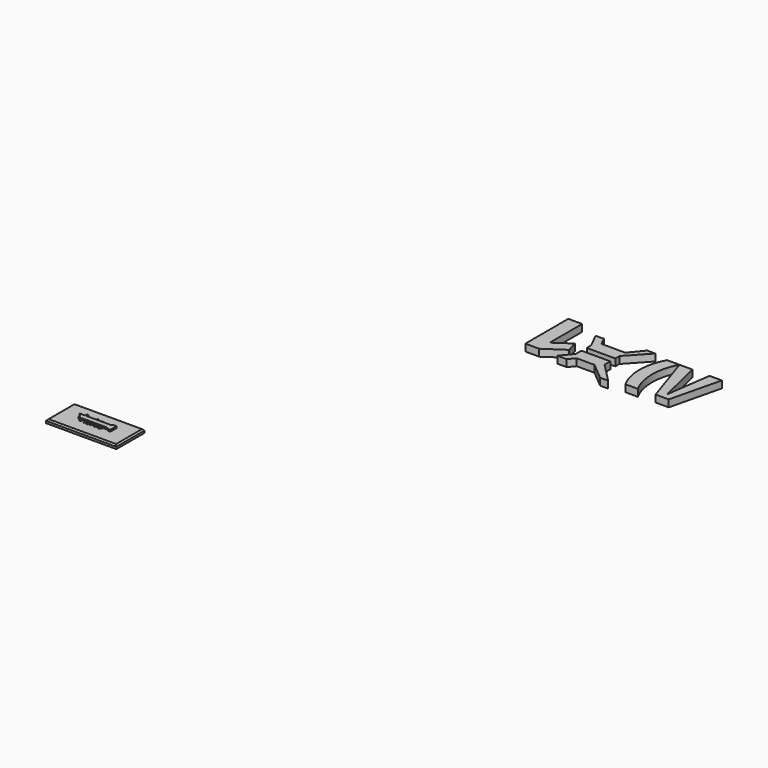
from build123d import *

# Parameters (mm, degrees)
F2_DEPTH      = 50.8
F0_W          = 208.8167369366
F0_H          = 51.5262037516
F0_W_2        = 205.8834665987
F0_H_2        = 38.4079218469
F4_DEPTH      = 50.8
F6_DEPTH      = 38.1
F7_W          = 508
F7_H          = 254
F8_DEPTH      = 25.4
F10_TEXT_SIZE = 24.7326162126
F9_TEXT_SIZE  = 38.4211540222
F11_DEPTH     = 25.4
F12_SIZE      = 10.16


# Not quite as in the source:
# - a feature names something its author has since deleted; it is built from what else it names
# - Text() gives the source's letters only with a copy of the font that has no kerning and outlines rounded to 1/6400 em; it was checked with that copy


with BuildPart() as f2:
    # F1 (on Top) → F2 (new body)
    with BuildSketch(Plane.XY):
        Polygon((1089.858174324, 166.3102060556), (997.6534247398, 166.3102060556), (1119.6892261505, -202.5089114904), (1214.6058082581, -202.5089114904), (1304.0987253189, 166.3102060556), (1214.6058082581, 166.3102060556), (1168.5034036636, -159.1184288263), align=None)
    extrude(amount=F2_DEPTH)


with BuildPart() as f2b:
    # F1 (on Top) → F2, piece 2 (new body)
    with BuildSketch(Plane.XY):
        with BuildLine():
            ThreePointArc((908.1605672836, 166.3102060556), (859.1155412482, -22.1672132611), (908.1605672836, -210.6446325779))
            Line((908.1605672836, -210.6446325779), (997.6534247398, -210.6446325779))
            ThreePointArc((997.6534247398, -210.6446325779), (949.8001223962, -22.1672132611), (997.6534247398, 166.3102060556))
            Line((997.6534247398, 166.3102060556), (908.1605672836, 166.3102060556))
        make_face()
    extrude(amount=F2_DEPTH)


with BuildPart() as f2c:
    # F0 (on Top) → F2, piece 3 (new body)
    with BuildSketch(Plane.XY):
        with Locations((562.3926073313, -70.981502533)):
            Rectangle(F0_W, F0_H)
        Polygon((666.8009757996, -96.7446044087), (457.984238863, -96.7446044087), (390.1866078377, -178.1017631292), (457.984238863, -178.1017631292), (494.6616488046, -134.0888703932), (623.4104633331, -134.0888703932), (747.2194167122, -237.2629963194), (805.1081299782, -237.2629963194), align=None)
    extrude(amount=F2_DEPTH)


with BuildPart() as f2d:
    # F0 (on Top) → F2, piece 4 (new body)
    with BuildSketch(Plane.XY):
        Polygon((406.4580502787, 147.3268717527), (460.9175092009, 38.4079218469), (666.8009757996, 38.4079218469), (805.1081299782, 188.0054622889), (747.2194167122, 188.0054622889), (666.8009757996, 90.376868844), (494.6616488046, 90.376868844), (466.1199748516, 147.3268717527), align=None)
        with Locations((563.8592425002, 19.2039609235)):
            Rectangle(F0_W_2, F0_H_2)
    extrude(amount=F2_DEPTH)


with BuildPart() as f4:
    # F3 (on Top) → F4 (new body)
    with BuildSketch(Plane.XY):
        Polygon((156.9627672434, 212.4126106501), (156.9627672434, -175.3898561001), (257.3032677174, -175.3898561001), (257.3032677174, -80.473177135), (257.3032677174, 212.4126106501), align=None)
        Polygon((257.3032677174, -80.473177135), (257.3032677174, -175.3898561001), (398.322314024, -80.473177135), (373.9151656628, 0), align=None)
    extrude(amount=F4_DEPTH)


with BuildPart() as f6:
    # F5 (on Top) → F6 (new body)
    with BuildSketch(Plane.XY):
        with BuildLine():
            Line((-1066.0594806806, -2393.8014631634), (-1240.2185239818, -2393.8014631634))
            Line((-1240.2185239818, -2393.8014631634), (-1240.2185239818, -2431.1765145333))
            Line((-1240.2185239818, -2431.1765145333), (-1066.0594806806, -2431.1765145333))
            Line((-1066.0594806806, -2431.1765145333), (-1061.7204306761, -2431.1765145333))
            ThreePointArc((-1061.7204306761, -2431.1765145333), (-1046.5276988746, -2440.3088155686), (-1028.8736676509, -2438.7109409353))
            Line((-1028.8736676509, -2438.7109409353), (-1028.8736676509, -2414.7824282699))
            Line((-1028.8736676509, -2414.7824282699), (-1028.8736676509, -2412.4889888483))
            Line((-1028.8736676509, -2412.4889888483), (-1028.8736676509, -2406.4367107859))
            Line((-1028.8736676509, -2406.4367107859), (-1028.8736676509, -2403.9940772423))
            Line((-1028.8736676509, -2403.9940772423), (-1028.8736676509, -2396.0567906488))
            Line((-1028.8736676509, -2396.0567906488), (-1028.8736676509, -2393.8014631634))
            Line((-1028.8736676509, -2393.8014631634), (-1028.8736676509, -2386.2670367614))
            ThreePointArc((-1028.8736676509, -2386.2670367614), (-1046.5276988746, -2384.6691621281), (-1061.7204306761, -2393.8014631634))
            Line((-1061.7204306761, -2393.8014631634), (-1066.0594806806, -2393.8014631634))
        make_face()
        Polygon((-1248.5956841506, -2430.5321082507), (-1248.5956841506, -2406.7832553444), (-1269.2164084326, -2406.7832553444), (-1269.2164084326, -2411.8445825658), align=None)
        Polygon((-1248.5956841506, -2406.7832553444), (-1248.5956841506, -2393.6926673954), (-1289.8371327145, -2393.1570568808), (-1269.2164084326, -2411.8445825658), (-1269.2164084326, -2406.7832553444), align=None)
        Polygon((-1240.2185239818, -2431.1765145333), (-1240.2185239818, -2393.8014631634), (-1248.5956841506, -2393.6926673954), (-1248.5956841506, -2406.7832553444), (-1248.5956841506, -2430.5321082507), (-1248.5956841506, -2445.9976430243), (-1240.2185239818, -2445.9976430243), align=None)
        Polygon((-1248.5956841506, -2393.6926673954), (-1240.2185239818, -2393.8014631634), (-1240.2185239818, -2376.4027230425), (-1248.5956841506, -2376.4027230425), align=None)
        Polygon((-1269.2164084326, -2430.5321082507), (-1248.5956841506, -2430.5321082507), (-1269.2164084326, -2411.8445825658), align=None)
    extrude(amount=F6_DEPTH)

    # F7 (on Top) → F8 (join)
    with BuildSketch(Plane.XY):
        with Locations((-1153.8031778336, -2421.0725765228)):
            Rectangle(F7_W, F7_H)
    extrude(amount=F8_DEPTH)

    # F10 (on face) + F9 (on face) → F11 (cut)
    with BuildSketch(Plane.XY.offset(25.4)):
        with Locations((-1217.7563905716, -2450.4928588867)):
            Text('Saber shop', F10_TEXT_SIZE, font='Open Sans', text_align=(TextAlign.LEFT, TextAlign.BOTTOM))
    with BuildSketch(Plane.XY.offset(25.4)):
        with Locations((-1186.7928504944, -2392.3490047455)):
            Text('Pro', F9_TEXT_SIZE, font='Open Sans', text_align=(TextAlign.LEFT, TextAlign.BOTTOM))
    extrude(amount=-F11_DEPTH, mode=Mode.SUBTRACT)

    # F12
    f12_edges = [f6.edges().sort_by_distance(p)[0] for p in [
        (-1153.803178, -2294.072577, 25.4),
        (-899.803178, -2421.072577, 25.4),
        (-1407.803178, -2421.072577, 25.4),
        (-1153.803178, -2548.072577, 25.4),
    ]]
    chamfer(f12_edges, length=F12_SIZE)


solid = Compound([f2.part, f2b.part, f2c.part, f2d.part, f4.part, f6.part])
